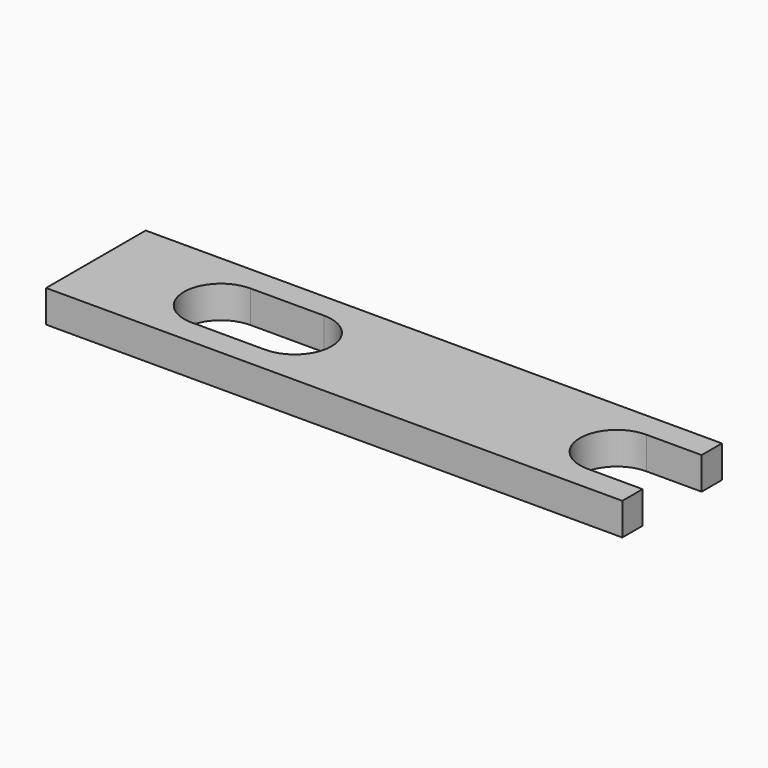
from build123d import *

# Parameters (mm, degrees)
F0_W     = 250
F0_H     = 27
F1_DEPTH = 7
F3_DEPTH = 25
F4_W     = 125
F4_H     = 94.8358140886
F5_DEPTH = 25


# Not quite as in the source:
# - ends of sketch curves that miss each other by under 0.0002 mm in the source are joined


with BuildPart() as f1:
    # F0 (on Top) → F1 (new body)
    with BuildSketch(Plane.XY):
        Rectangle(F0_W, F0_H)
    extrude(amount=F1_DEPTH)

    # F2 (on face) → F3 (cut)
    with BuildSketch(Plane.XY.offset(7)):
        with BuildLine():
            ThreePointArc((87, -8), (92.6568542495, -5.6568542495), (95, 0))
            ThreePointArc((95, 0), (92.6568542495, 5.6568542495), (87, 8))
            ThreePointArc((87, 8), (81.3431457505, 5.6568542495), (79, 0))
            ThreePointArc((79, 0), (81.3431457505, -5.6568542495), (87, -8))
        make_face()
        with BuildLine():
            ThreePointArc((79, 0), (81.3431457505, 5.6568542495), (87, 8))
            Line((87, 8), (71, 7.999994214))
            ThreePointArc((71, 7.999994214), (76.6568542495, 5.6568542495), (79, 0))
        make_face()
        with BuildLine():
            Line((71, -7.999994214), (87, -8))
            ThreePointArc((87, -8), (81.3431457505, -5.6568542495), (79, 0))
            ThreePointArc((79, 0), (76.6568542495, -5.6568542495), (71, -7.999994214))
        make_face()
        with BuildLine():
            ThreePointArc((71, -8), (76.6568542495, -5.6568542495), (79, 0))
            ThreePointArc((79, 0), (76.6568542495, 5.6568542495), (71, 8))
            ThreePointArc((71, 8), (63, 0), (71, -8))
        make_face()
        with BuildLine():
            ThreePointArc((-12, -8), (-6.3431457505, -5.6568542495), (-4, 0))
            ThreePointArc((-4, 0), (-6.3431457505, 5.6568542495), (-12, 8))
            ThreePointArc((-12, 8), (-20, 0), (-12, -8))
        make_face()
        with BuildLine():
            ThreePointArc((4, -8), (-1.6568542495, -5.6568542495), (-4, 0))
            ThreePointArc((-4, 0), (-6.3431457505, -5.6568542495), (-12, -8))
            Line((-12, -8), (4, -8))
        make_face()
        with BuildLine():
            ThreePointArc((-12, 8), (-6.3431457505, 5.6568542495), (-4, 0))
            ThreePointArc((-4, 0), (-1.6568542495, 5.6568542495), (4, 8))
            Line((4, 8), (-12, 8))
        make_face()
        with BuildLine():
            ThreePointArc((4, 8), (-1.6568542495, 5.6568542495), (-4, 0))
            ThreePointArc((-4, 0), (-1.6568542495, -5.6568542495), (4, -8))
            ThreePointArc((4, -8), (9.6568542495, -5.6568542495), (12, 0))
            ThreePointArc((12, 0), (9.6568542495, 5.6568542495), (4, 8))
        make_face()
        with BuildLine():
            ThreePointArc((-81.8808954364, -7.999994214), (-76.2178223077, -5.660255005), (-73.871273756, 0))
            ThreePointArc((-73.871273756, 0), (-76.2178223077, 5.660255005), (-81.8808954364, 7.999994214))
            Line((-81.8808954364, 7.999994214), (-81.8808954364, -7.999994214))
        make_face()
        with BuildLine():
            Line((-81.8808954364, -7.999994214), (-81.8808954364, 7.999994214))
            ThreePointArc((-81.8808954364, 7.999994214), (-87.531528761, 5.6534514483), (-89.871273756, 0))
            ThreePointArc((-89.871273756, 0), (-87.531528761, -5.6534514483), (-81.8808954364, -7.999994214))
        make_face()
        with BuildLine():
            ThreePointArc((-89.871273756, 0), (-87.531528761, 5.6534514483), (-81.8808954364, 7.999994214))
            Line((-81.8808954364, 7.999994214), (-97.871273756, 8))
            ThreePointArc((-97.871273756, 8), (-92.2144195065, 5.6568542495), (-89.871273756, 0))
        make_face()
        with BuildLine():
            Line((-97.32632471, -7.9814178275), (-81.8808954364, -7.999994214))
            ThreePointArc((-81.8808954364, -7.999994214), (-87.531528761, -5.6534514483), (-89.871273756, 0))
            ThreePointArc((-89.871273756, 0), (-92.0249247941, -5.4607878384), (-97.32632471, -7.9814178275))
        make_face()
        with BuildLine():
            ThreePointArc((-97.32632471, -7.9814178275), (-92.0249247941, -5.4607878384), (-89.871273756, 0))
            ThreePointArc((-89.871273756, 0), (-92.2144195065, 5.6568542495), (-97.871273756, 8))
            ThreePointArc((-97.871273756, 8), (-105.8662931823, 0.2822487793), (-98.4354198745, -7.9800839066))
            Line((-98.4354198745, -7.9800839066), (-97.32632471, -7.9814178275))
        make_face()
        with BuildLine():
            ThreePointArc((-98.4354198745, -7.9800839066), (-97.8808954364, -7.999994214), (-97.32632471, -7.9814178275))
            Line((-97.32632471, -7.9814178275), (-98.4354198745, -7.9800839066))
        make_face()
    extrude(amount=-F3_DEPTH, mode=Mode.SUBTRACT)

    # F4 (on face) → F5 (cut)
    with BuildSketch(Plane.XY.offset(7)):
        with Locations((62.5, -3.4542847425)):
            Rectangle(F4_W, F4_H)
    extrude(amount=-F5_DEPTH, mode=Mode.SUBTRACT)


solid = f1.part
